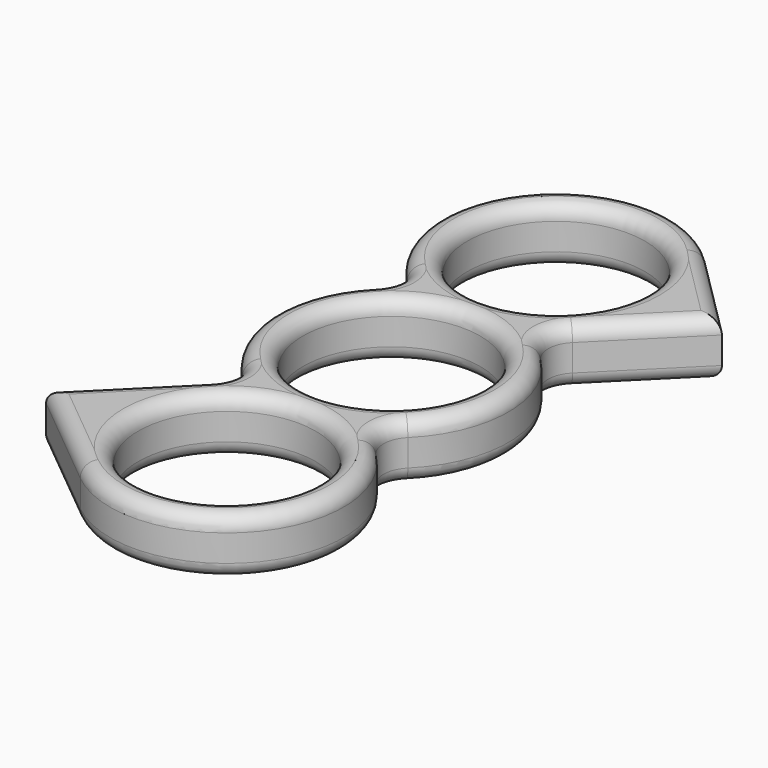
from build123d import *

# Parameters (mm, degrees)
F1_R         = 10.99185
F2_DEPTH     = 7
F3_T3_ANGLE  = 174.5093117662
F3_T6_ANGLE  = 90.1774978599
F3_T9_DEPTH  = 19.1358911422
F3_T12_DEPTH = 19.1358911422
F3_T15_ANGLE = 180
F3_T18_ANGLE = 90.1774978599
F3_T21_ANGLE = 90.1774978599
F3_T24_ANGLE = 90.1774978599
F3_T27_DEPTH = 20.6004844584
F3_T30_DEPTH = 20.6004844584
F3_T33_ANGLE = 90.1774978599
F3_T36_ANGLE = 90.1774978599
F3_T48_ANGLE = 90.1774978599
F3_T51_DEPTH = 19.1358911422
F3_T54_DEPTH = 19.1358911422
F3_T57_ANGLE = 180
F3_T60_ANGLE = 90.1774978599
F3_T63_ANGLE = 90.1774978599
F3_T66_ANGLE = 90.1774978599
F3_T69_DEPTH = 20.6004844584
F3_T72_DEPTH = 20.6004844584
F3_T75_ANGLE = 174.5093117662
F3_T78_ANGLE = 90.1774978599
F3_T81_ANGLE = 90.1774978599


# Not quite as in the source:
# - a fillet or chamfer that OpenCascade refuses, or shapes differently, is made with other operations: its cross-section is extruded or revolved along the edge and cut away or added


with BuildPart() as f2:
    # F1 (on Top) → F2 (new body)
    with BuildSketch(Plane.XY):
        with BuildLine():
            Line((20.5263900038, 25.4837), (10.2314004744, 35.7468457534))
            ThreePointArc((10.2314004744, 35.7468457534), (-10.2631457534, 35.7151004744), (-10.2314004744, 15.2205542466))
            ThreePointArc((-10.2314004744, 15.2205542466), (-9.2024377582, 12.74185), (-10.2314004744, 10.2631457534))
            ThreePointArc((-10.2314004744, 10.2631457534), (-14.49185, 0), (-10.2314004744, -10.2631457534))
            ThreePointArc((-10.2314004744, -10.2631457534), (-9.2024377582, -12.74185), (-10.2314004744, -15.2205542466))
            Line((-10.2314004744, -15.2205542466), (-21.5636167673, -26.5177184828))
            Line((-21.5636167673, -26.5177184828), (-9.2024377582, -36.6787371026))
            ThreePointArc((-9.2024377582, -36.6787371026), (10.7414195495, -35.2117842145), (10.2314004744, -15.2205542466))
            ThreePointArc((10.2314004744, -15.2205542466), (9.2024377582, -12.74185), (10.2314004744, -10.2631457534))
            ThreePointArc((10.2314004744, -10.2631457534), (14.49185, 0), (10.2314004744, 10.2631457534))
            ThreePointArc((10.2314004744, 10.2631457534), (9.2024377582, 12.74185), (10.2314004744, 15.2205542466))
            Line((10.2314004744, 15.2205542466), (20.5263900038, 25.4837))
        make_face()
        with Locations((0, -25.4837)):
            Circle(F1_R, mode=Mode.SUBTRACT)
        Circle(F1_R, mode=Mode.SUBTRACT)
        with Locations((0, 25.4837)):
            Circle(F1_R, mode=Mode.SUBTRACT)
    extrude(amount=F2_DEPTH)

    # F3: fillet of radius 1.8396307345 on 30 edges, made by hand


with BuildPart() as f3_tool1:
    # F3_s2 → F3_t3 (revolve)
    with BuildSketch(Plane(origin=(12.5009566595, -10.2759173125, 0), x_dir=(0, 0, 1), z_dir=(-0.7725057258, 0.635007798, 0))):
        with BuildLine():
            ThreePointArc((5.1603692655, -34.1781541649), (6.4611846327, -33.6393387977), (7, -32.3385234304))
            Line((7, -32.3385234304), (7, -34.1781541649))
            Line((7, -34.1781541649), (5.1603692655, -34.1781541649))
        make_face()
    revolve(axis=Axis((0, -25.4837, 7), (0, 0, 1)), revolution_arc=F3_T3_ANGLE)


with BuildPart() as f3_tool4:
    # F3_s5 → F3_t6 (revolve)
    with BuildSketch(Plane(origin=(0, 0, 0), x_dir=(0, 0, 1), z_dir=(0.7082012133, -0.7060106525, 0))):
        with BuildLine():
            ThreePointArc((5.1603692655, -14.49185), (6.4611846327, -13.9530346327), (7, -12.6522192655))
            Line((7, -12.6522192655), (7, -14.49185))
            Line((7, -14.49185), (5.1603692655, -14.49185))
        make_face()
    revolve(axis=Axis((12.7024377582, 12.74185, 7), (0, 0, -1)), revolution_arc=F3_T6_ANGLE)


with BuildPart() as f3_tool7:
    # F3_s8 → F3_t9 (new body)
    with BuildSketch(Plane(origin=(12.7417888575, 12.7023768048, 0), x_dir=(0, 0, 1), z_dir=(0.7082012133, 0.7060106525, 0))):
        with BuildLine():
            ThreePointArc((5.1603692655, -3.5557372601), (6.4611846327, -4.0945526273), (7, -5.3953679946))
            Line((7, -5.3953679946), (7, -3.5557372601))
            Line((7, -3.5557372601), (5.1603692655, -3.5557372601))
        make_face()
    extrude(amount=F3_T9_DEPTH)


with BuildPart() as f3_tool10:
    # F3_s11 → F3_t12 (new body)
    with BuildSketch(Plane(origin=(0.8102724675, -0.8077661867, 0), x_dir=(0, 0, 1), z_dir=(-0.7082012133, 0.7060106525, 0))):
        with BuildLine():
            ThreePointArc((5.1603692655, 32.5394372601), (6.4611846327, 32.0006218928), (7, 30.6998065255))
            Line((7, 30.6998065255), (7, 32.5394372601))
            Line((7, 32.5394372601), (5.1603692655, 32.5394372601))
        make_face()
    extrude(amount=F3_T12_DEPTH)


with BuildPart() as f3_tool13:
    # F3_s14 → F3_t15 (revolve)
    with BuildSketch(Plane(origin=(-12.7417888575, 12.7023768048, 0), x_dir=(0, 0, 1), z_dir=(0.7082012133, -0.7060106525, 0))):
        with BuildLine():
            ThreePointArc((5.1603692655, -32.5394372601), (6.4611846327, -32.0006218928), (7, -30.6998065255))
            Line((7, -30.6998065255), (7, -32.5394372601))
            Line((7, -32.5394372601), (5.1603692655, -32.5394372601))
        make_face()
    revolve(axis=Axis((0, 25.4837, 7), (0, 0, 1)), revolution_arc=F3_T15_ANGLE)


with BuildPart() as f3_tool16:
    # F3_s17 → F3_t18 (revolve)
    with BuildSketch(Plane(origin=(-12.7417888575, 12.7023768048, 0), x_dir=(0, 0, 1), z_dir=(-0.7082012133, 0.7060106525, 0))):
        with BuildLine():
            ThreePointArc((5.1603692655, 3.5557372601), (6.4611846327, 4.0945526273), (7, 5.3953679946))
            Line((7, 5.3953679946), (7, 3.5557372601))
            Line((7, 3.5557372601), (5.1603692655, 3.5557372601))
        make_face()
    revolve(axis=Axis((-12.7024377582, 12.74185, 7), (0, 0, -1)), revolution_arc=F3_T18_ANGLE)


with BuildPart() as f3_tool19:
    # F3_s20 → F3_t21 (revolve)
    with BuildSketch(Plane(origin=(0, 0, 0), x_dir=(0, 0, 1), z_dir=(0.7082012133, 0.7060106525, 0))):
        with BuildLine():
            ThreePointArc((5.1603692655, -14.49185), (6.4611846327, -13.9530346327), (7, -12.6522192655))
            Line((7, -12.6522192655), (7, -14.49185))
            Line((7, -14.49185), (5.1603692655, -14.49185))
        make_face()
    revolve(axis=Axis((0, 0, 7), (0, 0, 1)), revolution_arc=F3_T21_ANGLE)


with BuildPart() as f3_tool22:
    # F3_s23 → F3_t24 (revolve)
    with BuildSketch(Plane(origin=(0, 0, 0), x_dir=(0, 0, 1), z_dir=(-0.7082012133, 0.7060106525, 0))):
        with BuildLine():
            ThreePointArc((5.1603692655, -14.49185), (6.4611846327, -13.9530346327), (7, -12.6522192655))
            Line((7, -12.6522192655), (7, -14.49185))
            Line((7, -14.49185), (5.1603692655, -14.49185))
        make_face()
    revolve(axis=Axis((-12.7024377582, -12.74185, 7), (0, 0, -1)), revolution_arc=F3_T24_ANGLE)


with BuildPart() as f3_tool25:
    # F3_s26 → F3_t27 (new body)
    with BuildSketch(Plane(origin=(-12.7417888575, -12.7023768048, 0), x_dir=(0, 0, 1), z_dir=(-0.7082012133, -0.7060106525, 0))):
        with BuildLine():
            ThreePointArc((5.1603692655, -3.5557372601), (6.4611846327, -4.0945526273), (7, -5.3953679946))
            Line((7, -5.3953679946), (7, -3.5557372601))
            Line((7, -3.5557372601), (5.1603692655, -3.5557372601))
        make_face()
    extrude(amount=F3_T27_DEPTH)


with BuildPart() as f3_tool28:
    # F3_s29 → F3_t30 (new body)
    with BuildSketch(Plane(origin=(-3.4130355392, 2.8055509622, 0), x_dir=(0, 0, 1), z_dir=(0.7725057258, -0.635007798, 0))):
        with BuildLine():
            ThreePointArc((5.1603692655, 34.1781541649), (6.4611846327, 33.6393387977), (7, 32.3385234304))
            Line((7, 32.3385234304), (7, 34.1781541649))
            Line((7, 34.1781541649), (5.1603692655, 34.1781541649))
        make_face()
    extrude(amount=F3_T30_DEPTH)


with BuildPart() as f3_tool31:
    # F3_s32 → F3_t33 (revolve)
    with BuildSketch(Plane(origin=(12.7417888575, -12.7023768048, 0), x_dir=(0, 0, 1), z_dir=(0.7082012133, -0.7060106525, 0))):
        with BuildLine():
            ThreePointArc((5.1603692655, 3.5557372601), (6.4611846327, 4.0945526273), (7, 5.3953679946))
            Line((7, 5.3953679946), (7, 3.5557372601))
            Line((7, 3.5557372601), (5.1603692655, 3.5557372601))
        make_face()
    revolve(axis=Axis((12.7024377582, -12.74185, 7), (0, 0, -1)), revolution_arc=F3_T33_ANGLE)


with BuildPart() as f3_tool34:
    # F3_s35 → F3_t36 (revolve)
    with BuildSketch(Plane(origin=(0, 0, 0), x_dir=(0, 0, 1), z_dir=(-0.7082012133, -0.7060106525, 0))):
        with BuildLine():
            ThreePointArc((5.1603692655, -14.49185), (6.4611846327, -13.9530346327), (7, -12.6522192655))
            Line((7, -12.6522192655), (7, -14.49185))
            Line((7, -14.49185), (5.1603692655, -14.49185))
        make_face()
    revolve(axis=Axis((0, 0, 7), (0, 0, 1)), revolution_arc=F3_T36_ANGLE)


with BuildPart() as f3_tool37:
    # F3_s38 → F3_t39 (revolve)
    with BuildSketch(Plane.XZ.offset(25.4837)):
        with BuildLine():
            ThreePointArc((10.99185, 5.1603692655), (11.5306653673, 6.4611846327), (12.8314807345, 7))
            Line((12.8314807345, 7), (10.99185, 7))
            Line((10.99185, 7), (10.99185, 5.1603692655))
        make_face()
    revolve(axis=Axis((0, -25.4837, 7), (0, 0, 1)))


with BuildPart() as f3_tool40:
    # F3_s41 → F3_t42 (revolve)
    with BuildSketch(Plane.XZ):
        with BuildLine():
            ThreePointArc((10.99185, 5.1603692655), (11.5306653673, 6.4611846327), (12.8314807345, 7))
            Line((12.8314807345, 7), (10.99185, 7))
            Line((10.99185, 7), (10.99185, 5.1603692655))
        make_face()
    revolve(axis=Axis((0, 0, 7), (0, 0, 1)))


with BuildPart() as f3_tool43:
    # F3_s44 → F3_t45 (revolve)
    with BuildSketch(Plane.XZ.offset(-25.4837)):
        with BuildLine():
            ThreePointArc((10.99185, 5.1603692655), (11.5306653673, 6.4611846327), (12.8314807345, 7))
            Line((12.8314807345, 7), (10.99185, 7))
            Line((10.99185, 7), (10.99185, 5.1603692655))
        make_face()
    revolve(axis=Axis((0, 25.4837, 7), (0, 0, 1)))


with BuildPart() as f3_tool46:
    # F3_s47 → F3_t48 (revolve)
    with BuildSketch(Plane(origin=(0, 0, 0), x_dir=(0, 0, 1), z_dir=(0.7082012133, -0.7060106525, 0))):
        with BuildLine():
            ThreePointArc((1.8396307345, -14.49185), (0.5388153673, -13.9530346327), (0, -12.6522192655))
            Line((0, -12.6522192655), (0, -14.49185))
            Line((0, -14.49185), (1.8396307345, -14.49185))
        make_face()
    revolve(axis=Axis((12.7024377582, 12.74185, 0), (0, 0, -1)), revolution_arc=F3_T48_ANGLE)


with BuildPart() as f3_tool49:
    # F3_s50 → F3_t51 (new body)
    with BuildSketch(Plane(origin=(12.7417888575, 12.7023768048, 0), x_dir=(0, 0, 1), z_dir=(0.7082012133, 0.7060106525, 0))):
        with BuildLine():
            ThreePointArc((1.8396307345, -3.5557372601), (0.5388153673, -4.0945526273), (0, -5.3953679946))
            Line((0, -5.3953679946), (0, -3.5557372601))
            Line((0, -3.5557372601), (1.8396307345, -3.5557372601))
        make_face()
    extrude(amount=F3_T51_DEPTH)


with BuildPart() as f3_tool52:
    # F3_s53 → F3_t54 (new body)
    with BuildSketch(Plane(origin=(0.8102724675, -0.8077661867, 0), x_dir=(0, 0, 1), z_dir=(-0.7082012133, 0.7060106525, 0))):
        with BuildLine():
            ThreePointArc((1.8396307345, 32.5394372601), (0.5388153673, 32.0006218928), (0, 30.6998065255))
            Line((0, 30.6998065255), (0, 32.5394372601))
            Line((0, 32.5394372601), (1.8396307345, 32.5394372601))
        make_face()
    extrude(amount=F3_T54_DEPTH)


with BuildPart() as f3_tool55:
    # F3_s56 → F3_t57 (revolve)
    with BuildSketch(Plane(origin=(-12.7417888575, 12.7023768048, 0), x_dir=(0, 0, 1), z_dir=(0.7082012133, -0.7060106525, 0))):
        with BuildLine():
            ThreePointArc((1.8396307345, -32.5394372601), (0.5388153673, -32.0006218928), (0, -30.6998065255))
            Line((0, -30.6998065255), (0, -32.5394372601))
            Line((0, -32.5394372601), (1.8396307345, -32.5394372601))
        make_face()
    revolve(axis=Axis((0, 25.4837, 0), (0, 0, 1)), revolution_arc=F3_T57_ANGLE)


with BuildPart() as f3_tool58:
    # F3_s59 → F3_t60 (revolve)
    with BuildSketch(Plane(origin=(-12.7417888575, 12.7023768048, 0), x_dir=(0, 0, 1), z_dir=(-0.7082012133, 0.7060106525, 0))):
        with BuildLine():
            ThreePointArc((1.8396307345, 3.5557372601), (0.5388153673, 4.0945526273), (0, 5.3953679946))
            Line((0, 5.3953679946), (0, 3.5557372601))
            Line((0, 3.5557372601), (1.8396307345, 3.5557372601))
        make_face()
    revolve(axis=Axis((-12.7024377582, 12.74185, 0), (0, 0, -1)), revolution_arc=F3_T60_ANGLE)


with BuildPart() as f3_tool61:
    # F3_s62 → F3_t63 (revolve)
    with BuildSketch(Plane(origin=(0, 0, 0), x_dir=(0, 0, 1), z_dir=(0.7082012133, 0.7060106525, 0))):
        with BuildLine():
            ThreePointArc((1.8396307345, -14.49185), (0.5388153673, -13.9530346327), (0, -12.6522192655))
            Line((0, -12.6522192655), (0, -14.49185))
            Line((0, -14.49185), (1.8396307345, -14.49185))
        make_face()
    revolve(axis=Axis((0, 0, 0), (0, 0, 1)), revolution_arc=F3_T63_ANGLE)


with BuildPart() as f3_tool64:
    # F3_s65 → F3_t66 (revolve)
    with BuildSketch(Plane(origin=(0, 0, 0), x_dir=(0, 0, 1), z_dir=(-0.7082012133, 0.7060106525, 0))):
        with BuildLine():
            ThreePointArc((1.8396307345, -14.49185), (0.5388153673, -13.9530346327), (0, -12.6522192655))
            Line((0, -12.6522192655), (0, -14.49185))
            Line((0, -14.49185), (1.8396307345, -14.49185))
        make_face()
    revolve(axis=Axis((-12.7024377582, -12.74185, 0), (0, 0, -1)), revolution_arc=F3_T66_ANGLE)


with BuildPart() as f3_tool67:
    # F3_s68 → F3_t69 (new body)
    with BuildSketch(Plane(origin=(-12.7417888575, -12.7023768048, 0), x_dir=(0, 0, 1), z_dir=(-0.7082012133, -0.7060106525, 0))):
        with BuildLine():
            ThreePointArc((1.8396307345, -3.5557372601), (0.5388153673, -4.0945526273), (0, -5.3953679946))
            Line((0, -5.3953679946), (0, -3.5557372601))
            Line((0, -3.5557372601), (1.8396307345, -3.5557372601))
        make_face()
    extrude(amount=F3_T69_DEPTH)


with BuildPart() as f3_tool70:
    # F3_s71 → F3_t72 (new body)
    with BuildSketch(Plane(origin=(-3.4130355392, 2.8055509622, 0), x_dir=(0, 0, 1), z_dir=(0.7725057258, -0.635007798, 0))):
        with BuildLine():
            ThreePointArc((1.8396307345, 34.1781541649), (0.5388153673, 33.6393387977), (0, 32.3385234304))
            Line((0, 32.3385234304), (0, 34.1781541649))
            Line((0, 34.1781541649), (1.8396307345, 34.1781541649))
        make_face()
    extrude(amount=F3_T72_DEPTH)


with BuildPart() as f3_tool73:
    # F3_s74 → F3_t75 (revolve)
    with BuildSketch(Plane(origin=(12.5009566595, -10.2759173125, 0), x_dir=(0, 0, 1), z_dir=(-0.7725057258, 0.635007798, 0))):
        with BuildLine():
            ThreePointArc((1.8396307345, -34.1781541649), (0.5388153673, -33.6393387977), (0, -32.3385234304))
            Line((0, -32.3385234304), (0, -34.1781541649))
            Line((0, -34.1781541649), (1.8396307345, -34.1781541649))
        make_face()
    revolve(axis=Axis((0, -25.4837, 0), (0, 0, 1)), revolution_arc=F3_T75_ANGLE)


with BuildPart() as f3_tool76:
    # F3_s77 → F3_t78 (revolve)
    with BuildSketch(Plane(origin=(12.7417888575, -12.7023768048, 0), x_dir=(0, 0, 1), z_dir=(0.7082012133, -0.7060106525, 0))):
        with BuildLine():
            ThreePointArc((1.8396307345, 3.5557372601), (0.5388153673, 4.0945526273), (0, 5.3953679946))
            Line((0, 5.3953679946), (0, 3.5557372601))
            Line((0, 3.5557372601), (1.8396307345, 3.5557372601))
        make_face()
    revolve(axis=Axis((12.7024377582, -12.74185, 0), (0, 0, -1)), revolution_arc=F3_T78_ANGLE)


with BuildPart() as f3_tool79:
    # F3_s80 → F3_t81 (revolve)
    with BuildSketch(Plane(origin=(0, 0, 0), x_dir=(0, 0, 1), z_dir=(-0.7082012133, -0.7060106525, 0))):
        with BuildLine():
            ThreePointArc((1.8396307345, -14.49185), (0.5388153673, -13.9530346327), (0, -12.6522192655))
            Line((0, -12.6522192655), (0, -14.49185))
            Line((0, -14.49185), (1.8396307345, -14.49185))
        make_face()
    revolve(axis=Axis((0, 0, 0), (0, 0, 1)), revolution_arc=F3_T81_ANGLE)


with BuildPart() as f3_tool82:
    # F3_s83 → F3_t84 (revolve)
    with BuildSketch(Plane.XZ.offset(25.4837)):
        with BuildLine():
            ThreePointArc((10.99185, 1.8396307345), (11.5306653673, 0.5388153673), (12.8314807345, 0))
            Line((12.8314807345, 0), (10.99185, 0))
            Line((10.99185, 0), (10.99185, 1.8396307345))
        make_face()
    revolve(axis=Axis((0, -25.4837, 0), (0, 0, 1)))


with BuildPart() as f3_tool85:
    # F3_s86 → F3_t87 (revolve)
    with BuildSketch(Plane.XZ):
        with BuildLine():
            ThreePointArc((10.99185, 1.8396307345), (11.5306653673, 0.5388153673), (12.8314807345, 0))
            Line((12.8314807345, 0), (10.99185, 0))
            Line((10.99185, 0), (10.99185, 1.8396307345))
        make_face()
    revolve(axis=Axis((0, 0, 0), (0, 0, 1)))


with BuildPart() as f3_tool88:
    # F3_s89 → F3_t90 (revolve)
    with BuildSketch(Plane.XZ.offset(-25.4837)):
        with BuildLine():
            ThreePointArc((10.99185, 1.8396307345), (11.5306653673, 0.5388153673), (12.8314807345, 0))
            Line((12.8314807345, 0), (10.99185, 0))
            Line((10.99185, 0), (10.99185, 1.8396307345))
        make_face()
    revolve(axis=Axis((0, 25.4837, 0), (0, 0, 1)))


with BuildPart() as f2_1:
    add(f2.part)

    # F3_t91: cut F3_tool1, F3_tool4, F3_tool7, F3_tool10, F3_tool13, F3_tool16, F3_tool19, F3_tool22, F3_tool25, F3_tool28, F3_tool31, F3_tool34, F3_tool37, F3_tool40, F3_tool43, F3_tool46, F3_tool49, F3_tool52, F3_tool55, F3_tool58, F3_tool61, F3_tool64, F3_tool67, F3_tool70, F3_tool73, F3_tool76, F3_tool79, F3_tool82, F3_tool85, F3_tool88
    add([f3_tool1.part, f3_tool4.part, f3_tool7.part, f3_tool10.part, f3_tool13.part, f3_tool16.part, f3_tool19.part, f3_tool22.part, f3_tool25.part, f3_tool28.part, f3_tool31.part, f3_tool34.part, f3_tool37.part, f3_tool40.part, f3_tool43.part, f3_tool46.part, f3_tool49.part, f3_tool52.part, f3_tool55.part, f3_tool58.part, f3_tool61.part, f3_tool64.part, f3_tool67.part, f3_tool70.part, f3_tool73.part, f3_tool76.part, f3_tool79.part, f3_tool82.part, f3_tool85.part, f3_tool88.part], mode=Mode.SUBTRACT)


solid = f2_1.part
